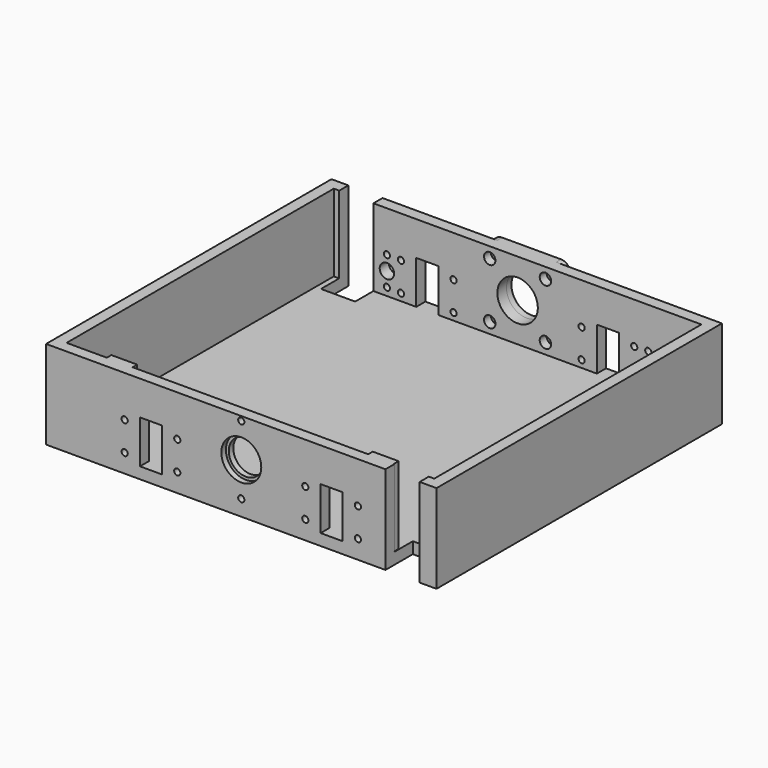
from build123d import *

# Parameters (mm, degrees)
F0_W      = 217.3440154
F0_H      = 198.6000092
F1_DEPTH  = 6.35
F2_W      = 217.3440154
F2_H      = 198.6000092
F2_W_2    = 204.6440154
F2_H_2    = 185.9000092
F3_DEPTH  = 43.0059846
F4_R      = 1.7272
F4_R_2    = 11.2530001
F4_R_3    = 4
F5_DEPTH  = 6.35
F6_DEPTH  = 6.35
F7_R      = 11.1125
F8_DEPTH  = 3.175
F9_R      = 9.525
F10_DEPTH = 3.175
F11_R     = 1.7272
F12_DEPTH = 6.35
F14_DEPTH = 3.175
F15_DEPTH = 3.175
F16_R     = 1.7272
F17_DEPTH = 6.35
F18_W     = 12.2546872
F18_H     = 24
F18_R     = 1.7272
F19_DEPTH = 198.6000092
F20_R     = 3.175
F21_DEPTH = 4.7625
F22_W     = 43.0059846
F22_H     = 43.0059846
F22_R     = 1.7272
F22_R_2   = 11.2530001
F23_DEPTH = 3.41249
F24_R     = 5.08
F25_W     = 19.05
F25_H     = 19.05
F26_DEPTH = 49.3559846


# Not quite as in the source:
# - a feature names something its author has since deleted; it is built from what else it names


with BuildPart() as f1:
    # F0 (on Top) → F1 (new body)
    with BuildSketch(Plane.XY):
        with Locations((108.6720077, -99.3000046)):
            Rectangle(F0_W, F0_H)
    extrude(amount=F1_DEPTH)

    # F2 (on face) → F3 (join)
    with BuildSketch(Plane.XY.offset(6.35)):
        with Locations((108.6720077, -99.3000046)):
            Rectangle(F2_W, F2_H)
        with Locations((108.6720077, -99.3000046)):
            Rectangle(F2_W_2, F2_H_2, mode=Mode.SUBTRACT)
    extrude(amount=F3_DEPTH)

    # F4 (on face) → F5 (cut, through all)
    with BuildSketch(Plane(origin=(0, 0, 0), x_dir=(-1, 0, 0), z_dir=(0, 1, 0))):
        with Locations((-124.1720021, 43.3529867)):
            Circle(F4_R)
        with Locations((-93.1720133, 43.3529867)):
            Circle(F4_R)
        with Locations((-124.1720021, 12.3529979)):
            Circle(F4_R)
        with Locations((-108.6720077, 27.8529923)):
            Circle(F4_R_2)
        with Locations((-93.1720133, 12.3529979)):
            Circle(F4_R)
        with Locations((-181.4220019, 18.6124977)):
            Circle(F4_R_3)
        with Locations((-35.9220135, 18.6124977)):
            Circle(F4_R_3)
    extrude(amount=-F5_DEPTH, mode=Mode.SUBTRACT)

    # F4 (on face) → F6 (cut, through all)
    with BuildSketch(Plane(origin=(0, 0, 0), x_dir=(-1, 0, 0), z_dir=(0, 1, 0))):
        with Locations((-124.1720021, 43.3529867)):
            Circle(F4_R)
        with Locations((-93.1720133, 43.3529867)):
            Circle(F4_R)
        with Locations((-124.1720021, 12.3529979)):
            Circle(F4_R)
        with Locations((-108.6720077, 27.8529923)):
            Circle(F4_R_2)
        with Locations((-93.1720133, 12.3529979)):
            Circle(F4_R)
        with Locations((-181.4220019, 18.6124977)):
            Circle(F4_R_3)
        with Locations((-35.9220135, 18.6124977)):
            Circle(F4_R_3)
    extrude(amount=-F6_DEPTH, mode=Mode.SUBTRACT)

    # F7 (on face) → F8 (cut)
    with BuildSketch(Plane.XZ.offset(198.6000092)):
        with Locations((108.6720077, 27.8529923)):
            Circle(F7_R)
    extrude(amount=-F8_DEPTH, mode=Mode.SUBTRACT)

    # F9 (on face) → F10 (cut, through all)
    with BuildSketch(Plane.XZ.offset(195.4250092)):
        with Locations((108.6720077, 27.8529923)):
            Circle(F9_R)
    extrude(amount=-F10_DEPTH, mode=Mode.SUBTRACT)

    # F11 (on face) → F12 (cut, through all)
    with BuildSketch(Plane.XZ.offset(198.6000092)):
        with Locations((108.6720077, 46.9029923)):
            Circle(F11_R)
        with Locations((108.6720077, 8.8029923)):
            Circle(F11_R)
    extrude(amount=-F12_DEPTH, mode=Mode.SUBTRACT)

    # F13 (on face) → F14 (join)
    with BuildSketch(Plane(origin=(0, -192.2500092, 0), x_dir=(-1, 0, 0), z_dir=(0, 1, 0))):
        Polygon((-28.7470088, 6.35), (-28.7470088, 49.3559846), (-35.9220135, 49.3559846), (-43.0970182, 49.3559846), (-43.0970182, 6.35), align=None)
        with BuildLine():
            ThreePointArc((-31.9220135, 18.6124977), (-38.7504406247, 15.7840705753), (-35.9220135, 22.6124977))
            ThreePointArc((-35.9220135, 22.6124977), (-33.0935863753, 21.4409248247), (-31.9220135, 18.6124977))
        make_face(mode=Mode.SUBTRACT)
        Polygon((-174.2469972, 6.35), (-174.2469972, 49.3559846), (-181.4220019, 49.3559846), (-188.5970066, 49.3559846), (-188.5970066, 6.35), align=None)
        with BuildLine():
            ThreePointArc((-177.4220019, 18.6124977), (-184.2504290247, 15.7840705753), (-181.4220019, 22.6124977))
            ThreePointArc((-181.4220019, 22.6124977), (-178.5935747753, 21.4409248247), (-177.4220019, 18.6124977))
        make_face(mode=Mode.SUBTRACT)
    extrude(amount=F14_DEPTH)

    # F15 (cut): faces of the model
    f15_faces = [f1.faces().sort_by_distance(p)[0] for p in [
        (181.4220019, -192.2500092, 18.6124977),
        (35.9220135, -192.2500092, 18.6124977),
    ]]
    extrude(f15_faces, amount=-F15_DEPTH, mode=Mode.SUBTRACT)

    # F16 (on face) → F17 (cut, through all)
    with BuildSketch(Plane(origin=(0, 0, 0), x_dir=(-1, 0, 0), z_dir=(0, 1, 0))):
        with Locations((-181.4220019, 10.6437477)):
            Circle(F16_R)
        with Locations((-181.4220019, 26.5812477)):
            Circle(F16_R)
        with Locations((-35.9220135, 10.6437477)):
            Circle(F16_R)
        with Locations((-35.9220135, 26.5812477)):
            Circle(F16_R)
    extrude(amount=-F17_DEPTH, mode=Mode.SUBTRACT)

    # F18 (on face) → F19 (cut, through all)
    with BuildSketch(Plane.XZ.offset(198.6000092)):
        with Locations((158.9532508, 18.35)):
            Rectangle(F18_W, F18_H)
        with Locations((173.5969985, 26.3812514)):
            Circle(F18_R)
        with Locations((173.5969985, 10.3187486)):
            Circle(F18_R)
        with Locations((144.3095031, 26.3812514)):
            Circle(F18_R)
        with Locations((144.3095031, 10.3187486)):
            Circle(F18_R)
        with Locations((58.3907646, 18.35)):
            Rectangle(F18_W, F18_H)
        with Locations((43.7470169, 26.3812514)):
            Circle(F18_R)
        with Locations((73.0345123, 26.3812514)):
            Circle(F18_R)
        with Locations((73.0345123, 10.3187486)):
            Circle(F18_R)
        with Locations((43.7470169, 10.3187486)):
            Circle(F18_R)
    extrude(amount=-F19_DEPTH, mode=Mode.SUBTRACT)

    # F20 (on face) → F21 (cut)
    with BuildSketch(Plane.XZ.offset(6.35)):
        with Locations((93.1720133, 43.3529867)):
            Circle(F20_R)
        with Locations((124.1720021, 43.3529867)):
            Circle(F20_R)
        with Locations((124.1720021, 12.3529979)):
            Circle(F20_R)
        with Locations((93.1720133, 12.3529979)):
            Circle(F20_R)
    extrude(amount=-F21_DEPTH, mode=Mode.SUBTRACT)

    # F22 (on face) → F23 (join)
    with BuildSketch(Plane(origin=(0, 0, 0), x_dir=(-1, 0, 0), z_dir=(0, 1, 0))):
        with Locations((-108.6720077, 27.8529923)):
            Rectangle(F22_W, F22_H)
        with Locations((-124.1720021, 12.3529979)):
            Circle(F22_R, mode=Mode.SUBTRACT)
        with Locations((-93.1720133, 12.3529979)):
            Circle(F22_R, mode=Mode.SUBTRACT)
        with Locations((-124.1720021, 43.3529867)):
            Circle(F22_R, mode=Mode.SUBTRACT)
        with Locations((-108.6720077, 27.8529923)):
            Circle(F22_R_2, mode=Mode.SUBTRACT)
        with Locations((-93.1720133, 43.3529867)):
            Circle(F22_R, mode=Mode.SUBTRACT)
    extrude(amount=F23_DEPTH)

    # F24
    f24_edges = [f1.edges().sort_by_distance(p)[0] for p in [
        (87.169015, 1.706245, 49.355985),
        (130.175, 1.706245, 49.355985),
        (87.169015, 1.706245, 6.35),
        (130.175, 1.706245, 6.35),
    ]]
    fillet(f24_edges, radius=F24_R)

    # F25 (on face) → F26 (cut, through all)
    with BuildSketch(Plane(origin=(0, 0, 0), x_dir=(1, 0, 0), z_dir=(0, 0, -1))):
        with Locations((198.4470123, 189.0750092)):
            Rectangle(F25_W, F25_H)
        with Locations((18.8970031, 9.525)):
            Rectangle(F25_W, F25_H)
    extrude(amount=-F26_DEPTH, mode=Mode.SUBTRACT)


solid = f1.part
